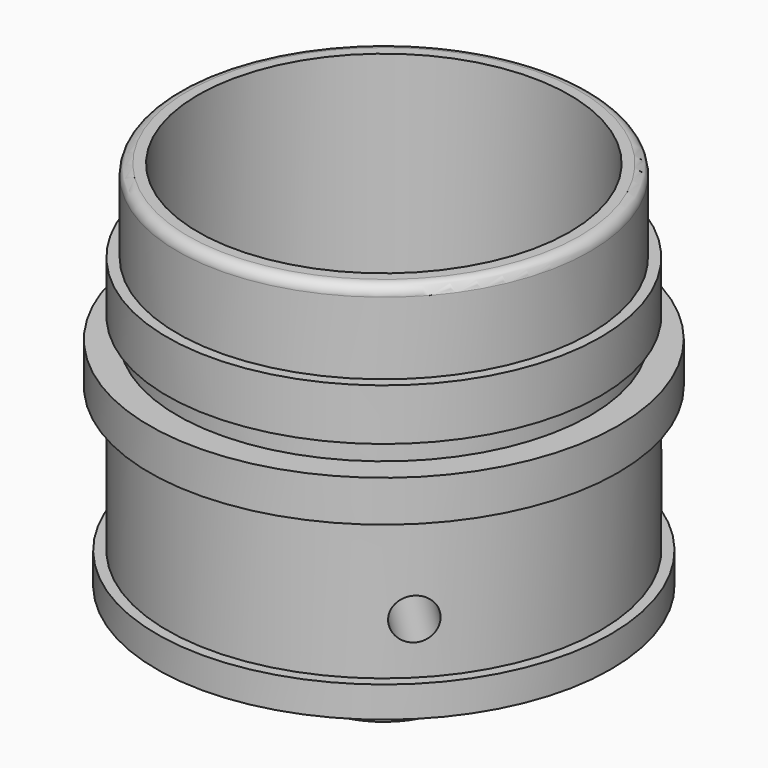
from build123d import *

# Parameters (mm, degrees)
F3_D           = 2.7
F3_CBORE_D     = 4.5
F3_CBORE_DEPTH = 3
F5_D           = 2.7
F5_DEPTH       = 3
F5_TIP         = 0.8111618357
F7_W           = 12.7133149276
F7_H           = 0.9999985352


# Not quite as in the source:
# - a pattern or mirror of a feature is missing from the dataset's text; its kind, count and spacing are read off the source's solid


with BuildPart() as f1:
    # F0 (on Front) → F1 (revolve)
    with BuildSketch(Plane.XZ):
        with BuildLine():
            Line((9.5, 22), (9, 22))
            Line((9, 22), (9, 12))
            Line((9, 12), (9.5, 11.5))
            Line((9.5, 11.5), (9.5, 10.5))
            Line((9.5, 10.5), (9, 10))
            Line((9, 10), (2, 10))
            Line((2, 10), (2, 6))
            Line((2, 6), (2.5, 6))
            Line((2.5, 6), (2.5, 0))
            Line((2.5, 0), (3.5, 0))
            Line((3.5, 0), (3.5, 3))
            Line((3.5, 3), (3.15, 3))
            Line((3.15, 3), (3.15, 4))
            Line((3.15, 4), (11, 4))
            Line((11, 4), (11, 5.5))
            Line((11, 5.5), (10.5, 5.5))
            Line((10.5, 5.5), (10.5, 12.5))
            Line((10.5, 12.5), (11.35, 12.5))
            Line((11.35, 12.5), (11.35, 14.5))
            Line((11.35, 14.5), (10, 14.5))
            Line((10, 14.5), (10, 15.5))
            Line((10, 15.5), (10.5, 15.5))
            Line((10.5, 15.5), (10.5, 18))
            Line((10.5, 18), (10, 18))
            Line((10, 18), (10, 21.5))
            ThreePointArc((10, 21.5), (9.8535533906, 21.8535533906), (9.5, 22))
        make_face()
    revolve(axis=Axis((0, 0, 11), (0, 0, 1)))

    # F3 (through all)
    with Locations(Plane(origin=(0, 0, 4), x_dir=(1, 0, 0), z_dir=(0, 0, -1))):
        with Locations((0, -5.75), (0, 5.75)):
            CounterBoreHole(F3_D / 2, F3_CBORE_D / 2, F3_CBORE_DEPTH)

    # F5
    with Locations(Plane.XY.offset(10)):
        with Locations((3, -3), (3, 3)):
            Hole(F5_D / 2, depth=F5_DEPTH)
            with Locations((0, 0, -(F5_DEPTH + F5_TIP / 2))):  # 118° drill point
                Cone(0, F5_D / 2, F5_TIP, mode=Mode.SUBTRACT)

    # F7 (on face) → F8 (revolve, cut)
    with BuildSketch(Plane(origin=(0, 0, 0), x_dir=(-0.7071067812, -0.7071067812, 0), z_dir=(-0.7071067812, 0.7071067812, 0))):
        with Locations((-10.5992981509, 8.4999992676)):
            Rectangle(F7_W, F7_H)
    f8 = revolve(axis=Axis((7.4948355983, 7.4948355983, 8), (0.7071067812, 0.7071067812, 0)), mode=Mode.SUBTRACT)

    # F8_copies: F8 across plane
    add(f8.mirror(Plane(origin=(0, -1.1e-05, 0), x_dir=(-1, -1e-06, 0), z_dir=(1e-06, -1, 0))), mode=Mode.SUBTRACT)


solid = f1.part
